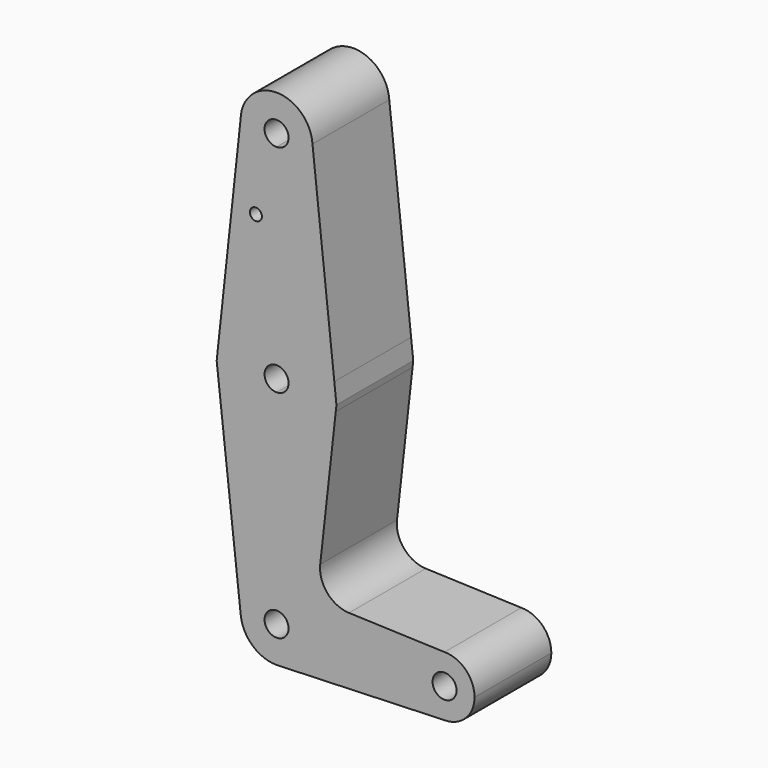
from build123d import *

# Parameters (mm, degrees)
F0_R     = 1.5875
F1_DEPTH = 25.4


with BuildPart() as f1:
    # F0 (on Front) → F1 (new body)
    with BuildSketch(Plane.XZ):
        with BuildLine():
            ThreePointArc((-44.9749847751, 74.0057436376), (-42.239710519, 67.1728704693), (-35.4511886835, 64.3293071628))
            ThreePointArc((-35.4511886835, 64.3293071628), (-28.7159965927, 67.119115072), (-25.9261886835, 73.8543071628))
            ThreePointArc((-25.9261886835, 73.8543071628), (-25.931047818, 74.1585158089), (-25.9456202636, 74.4624140737))
            ThreePointArc((-25.9456202636, 74.4624140737), (-35.6797057153, 83.3765655591), (-44.9749847751, 74.0057436376))
        make_face()
        with BuildLine():
            ThreePointArc((-32.2761886835, 73.8543071628), (-33.2061246532, 71.6092431325), (-35.4511886835, 70.6793071628))
            ThreePointArc((-35.4511886835, 70.6793071628), (-37.6962527138, 76.099371193), (-32.2761886835, 73.8543071628))
        make_face(mode=Mode.SUBTRACT)
        with BuildLine():
            ThreePointArc((-25.9261886835, 73.8543071628), (-28.7159965927, 67.119115072), (-35.4511886835, 64.3293071628))
            Line((-35.4511886835, 64.3293071628), (-35.4511886835, 32.5793071628))
            ThreePointArc((-35.4511886835, 32.5793071628), (-25.8667813668, 29.3595338058), (-20.1702001062, 21.0062849753))
            Line((-20.1702001062, 21.0062849753), (-25.9456202636, 74.4624140737))
            ThreePointArc((-25.9456202636, 74.4624140737), (-25.931047818, 74.1585158089), (-25.9261886835, 73.8543071628))
        make_face()
        with BuildLine():
            Line((-35.4511886835, 32.5793071628), (-35.4511886835, 64.3293071628))
            ThreePointArc((-35.4511886835, 64.3293071628), (-42.239710519, 67.1728704693), (-44.9749847751, 74.0057436376))
            Line((-44.9749847751, 74.0057436376), (-50.7276259168, 21.0224190715))
            ThreePointArc((-50.7276259168, 21.0224190715), (-45.0289127986, 29.3645925377), (-35.4511886835, 32.5793071628))
        make_face()
        with Locations((-40.9250855446, 53.2295071628)):
            Circle(F0_R, mode=Mode.SUBTRACT)
        with BuildLine():
            ThreePointArc((-20.1702001062, 21.0062849753), (-25.8667813668, 29.3595338058), (-35.4511886835, 32.5793071628))
            Line((-35.4511886835, 32.5793071628), (-35.4511886835, 19.8793071628))
            ThreePointArc((-35.4511886835, 19.8793071628), (-33.2061246532, 18.949371193), (-32.2761886835, 16.7043071628))
            ThreePointArc((-32.2761886835, 16.7043071628), (-33.2061246532, 14.4592431325), (-35.4511886835, 13.5293071628))
            Line((-35.4511886835, 13.5293071628), (-35.4511886835, 0.8293071628))
            ThreePointArc((-35.4511886835, 0.8293071628), (-25.1755047485, 4.6036483101), (-19.7859860662, 14.131944055))
            Line((-19.7859860662, 14.131944055), (-19.6039763716, 15.7654318029))
            Line((-19.6039763716, 15.7654318029), (-20.1702001062, 21.0062849753))
        make_face()
        with BuildLine():
            Line((-35.4511886835, 19.8793071628), (-35.4511886835, 32.5793071628))
            ThreePointArc((-35.4511886835, 32.5793071628), (-45.0289127986, 29.3645925377), (-50.7276259168, 21.0224190715))
            Line((-50.7276259168, 21.0224190715), (-51.2984009954, 15.7654318029))
            Line((-51.2984009954, 15.7654318029), (-51.1163913008, 14.131944055))
            ThreePointArc((-51.1163913008, 14.131944055), (-45.7268726185, 4.6036483101), (-35.4511886835, 0.8293071628))
            Line((-35.4511886835, 0.8293071628), (-35.4511886835, 13.5293071628))
            ThreePointArc((-35.4511886835, 13.5293071628), (-38.6261886835, 16.7043071628), (-35.4511886835, 19.8793071628))
        make_face()
        with BuildLine():
            ThreePointArc((-19.7859860662, 14.131944055), (-25.1755047485, 4.6036483101), (-35.4511886835, 0.8293071628))
            Line((-35.4511886835, 0.8293071628), (-35.4511886835, -30.9206928372))
            ThreePointArc((-35.4511886835, -30.9206928372), (-28.7159965927, -33.7105007464), (-25.9261886835, -40.4456928372))
            Line((-25.9261886835, -40.4456928372), (1.0613113165, -40.4456928372))
            ThreePointArc((1.0613113165, -40.4456928372), (3.3861512408, -34.8330327616), (8.9988113165, -32.5081928372))
            Line((8.9988113165, -32.5081928372), (-16.2812915947, -31.605332019))
            ThreePointArc((-16.2812915947, -31.605332019), (-22.0159487809, -28.8548482736), (-23.8988395601, -22.7798029084))
            Line((-23.8988395601, -22.7798029084), (-19.7859860662, 14.131944055))
        make_face()
        with BuildLine():
            Line((-35.4511886835, -30.9206928372), (-35.4511886835, 0.8293071628))
            ThreePointArc((-35.4511886835, 0.8293071628), (-45.7268726185, 4.6036483101), (-51.1163913008, 14.131944055))
            Line((-51.1163913008, 14.131944055), (-44.9176057417, -41.5004786351))
            ThreePointArc((-44.9176057417, -41.5004786351), (-42.5495145328, -34.0943626508), (-35.4511886835, -30.9206928372))
        make_face()
        with BuildLine():
            ThreePointArc((-25.9261886835, -40.4456928372), (-28.7159965927, -33.7105007464), (-35.4511886835, -30.9206928372))
            Line((-35.4511886835, -30.9206928372), (-35.4511886835, -37.2706928372))
            ThreePointArc((-35.4511886835, -37.2706928372), (-33.2061246532, -38.200628807), (-32.2761886835, -40.4456928372))
            Line((-32.2761886835, -40.4456928372), (-25.9261886835, -40.4456928372))
        make_face()
        with BuildLine():
            Line((-35.4511886835, -37.2706928372), (-35.4511886835, -30.9206928372))
            ThreePointArc((-35.4511886835, -30.9206928372), (-42.5495145328, -34.0943626508), (-44.9176057417, -41.5004786351))
            ThreePointArc((-44.9176057417, -41.5004786351), (-41.80251887, -47.5440186865), (-35.4511886835, -49.9706928372))
            Line((-35.4511886835, -49.9706928372), (-34.7716982376, -49.9464253213))
            ThreePointArc((-34.7716982376, -49.9464253213), (-28.4798985771, -46.9362043157), (-25.9261886835, -40.4456928372))
            Line((-25.9261886835, -40.4456928372), (-32.2761886835, -40.4456928372))
            ThreePointArc((-32.2761886835, -40.4456928372), (-37.6962527138, -42.6907568675), (-35.4511886835, -37.2706928372))
        make_face()
        with BuildLine():
            Line((1.0613113165, -40.4456928372), (-25.9261886835, -40.4456928372))
            ThreePointArc((-25.9261886835, -40.4456928372), (-28.4798985771, -46.9362043157), (-34.7716982376, -49.9464253213))
            Line((-34.7716982376, -49.9464253213), (8.9988113165, -48.3831928372))
            ThreePointArc((8.9988113165, -48.3831928372), (3.3861512408, -46.0583529129), (1.0613113165, -40.4456928372))
        make_face()
        with BuildLine():
            ThreePointArc((8.9988113165, -32.5081928372), (3.3861512408, -34.8330327616), (1.0613113165, -40.4456928372))
            ThreePointArc((1.0613113165, -40.4456928372), (3.3861512408, -46.0583529129), (8.9988113165, -48.3831928372))
            ThreePointArc((8.9988113165, -48.3831928372), (14.6114713922, -46.0583529129), (16.9363113165, -40.4456928372))
            ThreePointArc((16.9363113165, -40.4456928372), (14.6114713922, -34.8330327616), (8.9988113165, -32.5081928372))
        make_face()
        with BuildLine():
            ThreePointArc((12.1738113165, -40.4456928372), (8.9988113165, -43.6206928372), (5.8238113165, -40.4456928372))
            ThreePointArc((5.8238113165, -40.4456928372), (8.9988113165, -37.2706928372), (12.1738113165, -40.4456928372))
        make_face(mode=Mode.SUBTRACT)
    extrude(amount=F1_DEPTH)


solid = f1.part
